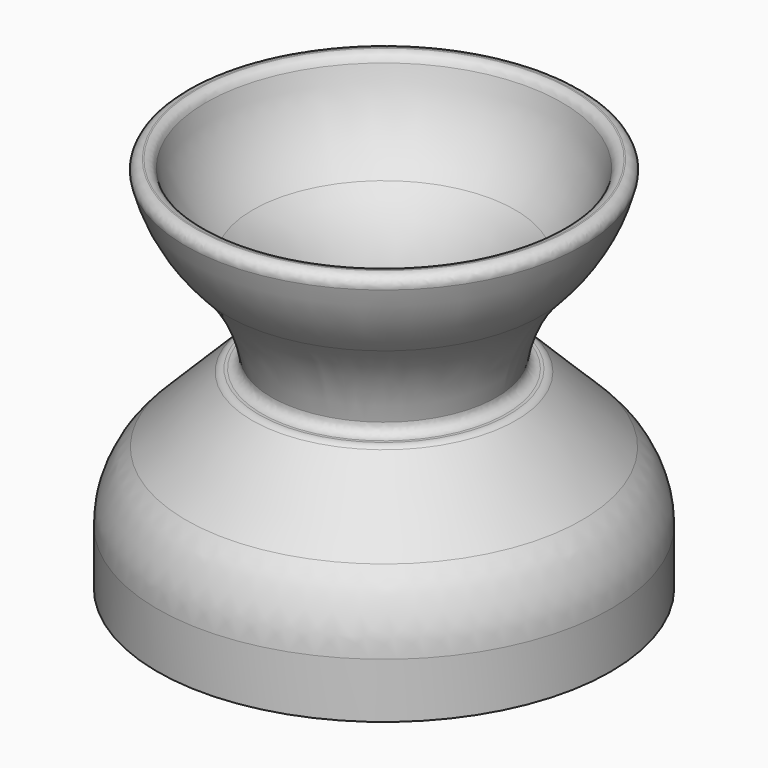
from build123d import *

# Parameters (mm, degrees)
F2_SIZE = 25.4
F3_R    = 2.54
F4_R    = 2.54
F5_R    = 25.4


with BuildPart() as f1:
    # F0 (on Front) → F1 (revolve)
    with BuildSketch(Plane.XZ):
        with BuildLine():
            Line((-54.2157366872, 0), (0, 0))
            Line((0, 0), (0, 6.5787681378))
            Line((0, 6.5787681378), (-53.7426385557, 6.5787681378))
            ThreePointArc((-53.7426385557, 6.5787681378), (-43.7672480582, 29.182630018), (-23.5321354121, 43.3594845235))
            Line((-23.5321354121, 43.3594845235), (-23.5321354121, 50.283357501))
            Line((-23.5321354121, 50.283357501), (-28.9389695972, 50.283357501))
            Line((-28.9389695972, 50.283357501), (-58.9924529195, 50.283357501))
            Line((-58.9924529195, 50.283357501), (-58.9924529195, 43.3594845235))
            Line((-58.9924529195, 43.3594845235), (-58.9924529195, 6.5787681378))
            Line((-58.9924529195, 6.5787681378), (-58.9924529195, 0))
            Line((-58.9924529195, 0), (-54.2157366872, 0))
        make_face()
        with BuildLine():
            Line((-28.9389695972, 50.283357501), (-23.5321354121, 50.283357501))
            ThreePointArc((-23.5321354121, 50.283357501), (-26.2905849886, 63.9954671693), (-34.1367754588, 75.5742534064))
            ThreePointArc((-34.1367754588, 75.5742534064), (-42.5334894353, 85.7479701823), (-46.6347932816, 98.285458982))
            Line((-46.6347932816, 98.285458982), (-52.2693172097, 98.285458982))
            ThreePointArc((-52.2693172097, 98.285458982), (-48.2156517017, 86.0893655487), (-40.8258400857, 75.5742534064))
            ThreePointArc((-40.8258400857, 75.5742534064), (-32.6149356607, 63.9945293644), (-28.9389695972, 50.283357501))
        make_face()
    revolve(axis=Axis((0, 0, 3.2893840689), (0, 0, 1)))

    # F2
    f2_edges = [f1.edges().sort_by_distance(p)[0] for p in [
        (58.992453, 0, 50.283358),
    ]]
    chamfer(f2_edges, length=F2_SIZE)

    # F3
    f3_edges = [f1.edges().sort_by_distance(p)[0] for p in [
        (33.592453, 0, 50.283358),
        (28.93897, 0, 50.283358),
    ]]
    fillet(f3_edges, radius=F3_R)

    # F4
    f4_edges = [f1.edges().sort_by_distance(p)[0] for p in [
        (46.634793, 0, 98.285459),
        (52.269317, 0, 98.285459),
    ]]
    fillet(f4_edges, radius=F4_R)

    # F5
    f5_edges = [f1.edges().sort_by_distance(p)[0] for p in [
        (58.992453, 0, 24.883358),
    ]]
    fillet(f5_edges, radius=F5_R)


solid = f1.part
